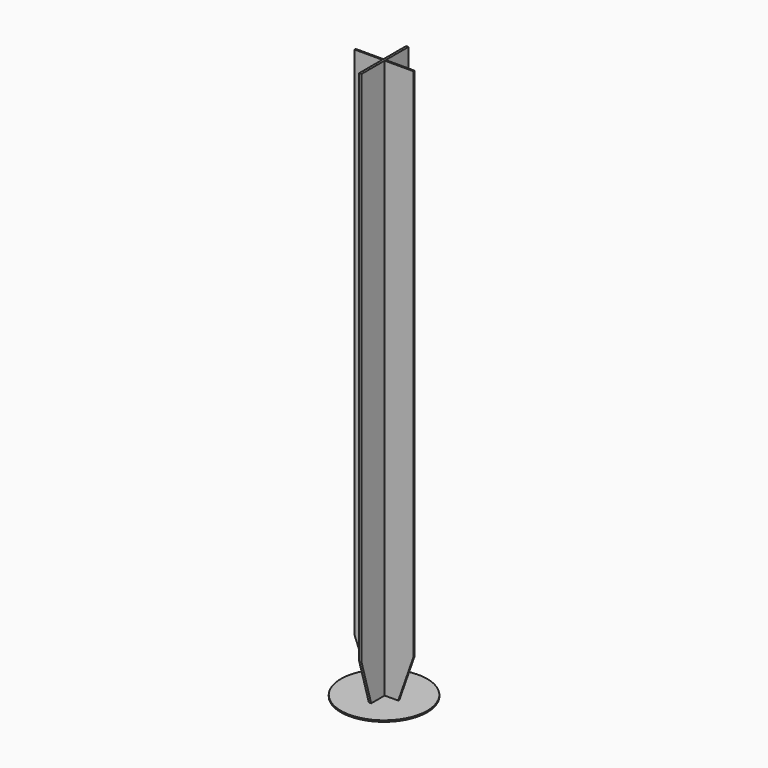
from build123d import *

# Parameters (mm, degrees)
F0_R     = 9.25
F3_DEPTH = 0.3
F4_DEPTH = 0.25
F5_DEPTH = 0.15


with BuildPart() as f3:
    # F0 (on Top) → F3 (new body)
    with BuildSketch(Plane.XY):
        Circle(F0_R)
    extrude(amount=F3_DEPTH)


with BuildPart() as f4:
    # F1 (on Right) → F4 (new body, symmetric)
    with BuildSketch(Plane.YZ):
        Polygon((-6.3975099474, 9.3173701316), (-3.669354599, 0), (2.6220979635, 0), (6.2024900526, 9.4951791689), (6.2024900526, 120), (-6.3975099474, 120), align=None)
    extrude(amount=F4_DEPTH, both=True)

    # F2 (on Front) → F5 (join, symmetric)
    with BuildSketch(Plane.XZ):
        Polygon((-6.1816425862, 9.5772715285), (-2.373900963, 0), (3.051972948, 0), (6.4183574138, 9.5772715285), (6.4183574138, 120), (-6.1816425862, 120), align=None)
    extrude(amount=F5_DEPTH, both=True)


solid = Compound([f3.part, f4.part])
